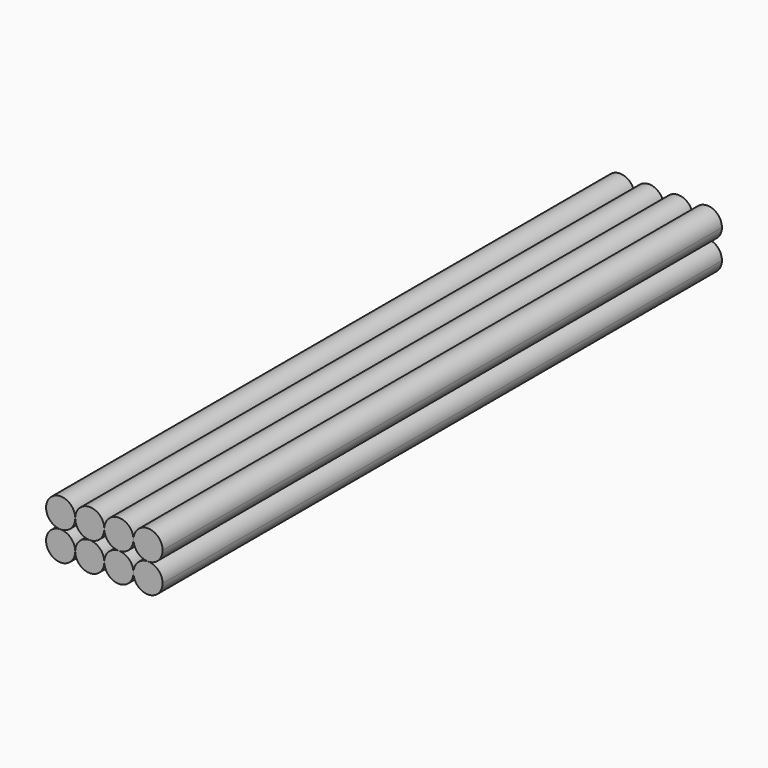
from build123d import *

# Parameters (mm, degrees)
F1_DEPTH = 121.92


with BuildPart() as f1:
    # F0 (on Front) → F1 (new body)
    with BuildSketch(Plane.XZ):
        with BuildLine():
            ThreePointArc((0, 2.54), (-1.7960512242, -1.7960512242), (2.54, 0))
            ThreePointArc((2.54, 0), (1.7960512242, 1.7960512242), (0, 2.54))
        make_face()
    extrude(amount=F1_DEPTH)


with BuildPart() as f1b:
    # F0 (on Front) → F1, piece 2 (new body)
    with BuildSketch(Plane.XZ):
        with BuildLine():
            ThreePointArc((2.54, 5.08), (-1.7960512242, 6.8760512242), (0, 2.54))
            ThreePointArc((0, 2.54), (1.7960512242, 3.2839487758), (2.54, 5.08))
        make_face()
    extrude(amount=F1_DEPTH)


with BuildPart() as f1c:
    # F0 (on Front) → F1, piece 3 (new body)
    with BuildSketch(Plane.XZ):
        with BuildLine():
            ThreePointArc((15.2399545881, 2.577204187), (13.4395241733, 1.828865517), (12.6999848625, 0.0248028653))
            ThreePointArc((12.6999848625, 0.0248028653), (15.2461552675, -2.5027882444), (17.7799545881, 0.037204187))
            ThreePointArc((17.7799545881, 0.037204187), (17.0360058124, 1.8332554112), (15.2399545881, 2.577204187))
        make_face()
    extrude(amount=F1_DEPTH)


with BuildPart() as f1d:
    # F0 (on Front) → F1, piece 4 (new body)
    with BuildSketch(Plane.XZ):
        with BuildLine():
            ThreePointArc((12.6999848625, 5.1048028653), (13.4482932582, 3.3167737722), (15.2399545881, 2.577204187))
            ThreePointArc((15.2399545881, 2.577204187), (17.0360058124, 3.3211529628), (17.7799545881, 5.117204187))
            ThreePointArc((17.7799545881, 5.117204187), (15.2337539088, 7.6571966184), (12.6999848625, 5.1048028653))
        make_face()
    extrude(amount=F1_DEPTH)


with BuildPart() as f1e:
    # F0 (on Front) → F1, piece 5 (new body)
    with BuildSketch(Plane.XZ):
        with BuildLine():
            ThreePointArc((5.0799848627, 2.5524013957), (3.2795544479, 1.8040627257), (2.5400151371, 7.39e-08))
            ThreePointArc((2.5400151371, 7.39e-08), (5.0861855421, -2.5275910357), (7.6199848627, 0.0124013957))
            ThreePointArc((7.6199848627, 0.0124013957), (6.8760360869, 1.8084526199), (5.0799848627, 2.5524013957))
        make_face()
    extrude(amount=F1_DEPTH)


with BuildPart() as f1f:
    # F0 (on Front) → F1, piece 6 (new body)
    with BuildSketch(Plane.XZ):
        with BuildLine():
            ThreePointArc((2.5400151371, 5.0800000739), (3.2883235327, 3.2919709808), (5.0799848627, 2.5524013957))
            ThreePointArc((5.0799848627, 2.5524013957), (6.8760360869, 3.2963501715), (7.6199848627, 5.0924013957))
            ThreePointArc((7.6199848627, 5.0924013957), (5.0737841834, 7.6323938271), (2.5400151371, 5.0800000739))
        make_face()
    extrude(amount=F1_DEPTH)


with BuildPart() as f1g:
    # F0 (on Front) → F1, piece 7 (new body)
    with BuildSketch(Plane.XZ):
        with BuildLine():
            ThreePointArc((10.1599697254, 2.5648027913), (8.3595393106, 1.8164641213), (7.6199999998, 0.0124014696))
            ThreePointArc((7.6199999998, 0.0124014696), (10.1661704048, -2.5151896401), (12.6999697254, 0.0248027913))
            ThreePointArc((12.6999697254, 0.0248027913), (11.9560209496, 1.8208540156), (10.1599697254, 2.5648027913))
        make_face()
    extrude(amount=F1_DEPTH)


with BuildPart() as f1h:
    # F0 (on Front) → F1, piece 8 (new body)
    with BuildSketch(Plane.XZ):
        with BuildLine():
            ThreePointArc((7.6199999998, 5.0924014696), (8.3683083954, 3.3043723765), (10.1599697254, 2.5648027913))
            ThreePointArc((10.1599697254, 2.5648027913), (11.9560209496, 3.3087515671), (12.6999697254, 5.1048027913))
            ThreePointArc((12.6999697254, 5.1048027913), (10.1537690461, 7.6447952228), (7.6199999998, 5.0924014696))
        make_face()
    extrude(amount=F1_DEPTH)


solid = Compound([f1.part, f1b.part, f1c.part, f1d.part, f1e.part, f1f.part, f1g.part, f1h.part])
